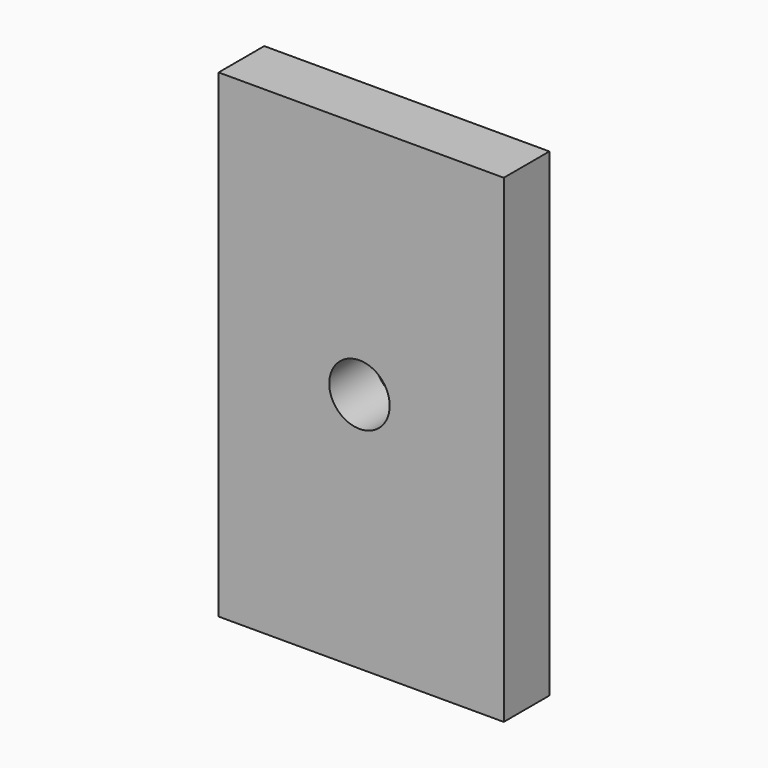
from build123d import *

# Parameters (mm, degrees)
F1_DEPTH = 3.175
F2_R     = 1.68275
F3_DEPTH = 3.176


# Not quite as in the source:
# - a feature names something its author has since deleted; it is built from what else it names


with BuildPart() as f1:
    # F0 (on Front) → F1 (new body)
    with BuildSketch(Plane.XZ):
        Polygon((9.525, 11.43), (9.525, 38.1), (-6.35, 38.1), (-6.35, 29.21), (-6.35, 20.32), (-6.35, 11.43), align=None)
    extrude(amount=F1_DEPTH)

    # F2 (on face) → F3 (cut, through all)
    with BuildSketch(Plane.XZ.offset(3.175)):
        with Locations((1.49225, 24.86025)):
            Circle(F2_R)
    extrude(amount=-F3_DEPTH, mode=Mode.SUBTRACT)


solid = f1.part
